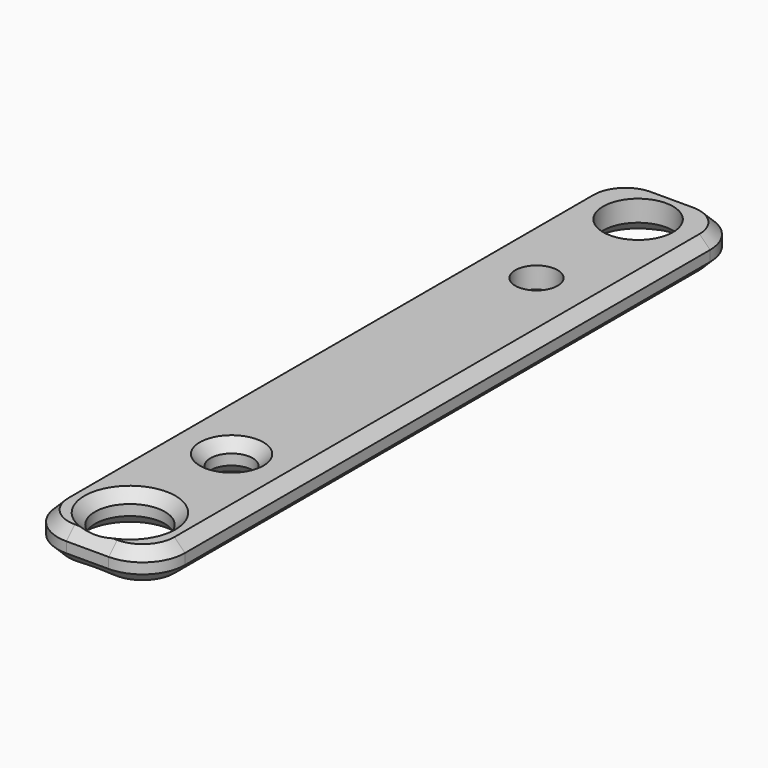
from build123d import *

# Parameters (mm, degrees)
F0_W         = 6
F0_H         = 35
F0_R         = 1.65
F0_R_2       = 1
F1_DEPTH     = 1.5
F2_R         = 2
F3_T1_DEPTH  = 31
F3_T3_DEPTH  = 2
F3_T6_ANGLE  = 90
F3_T8_ANGLE  = 90
F3_T10_ANGLE = 90
F3_T12_ANGLE = 90
F3_T14_ANGLE = 90
F3_T16_ANGLE = 90
F3_T18_ANGLE = 90
F3_T20_ANGLE = 90


# Not quite as in the source:
# - a fillet or chamfer that OpenCascade refuses, or shapes differently, is made with other operations: its cross-section is extruded or revolved along the edge and cut away or added


with BuildPart() as f1:
    # F0 (on Top) → F1 (new body)
    with BuildSketch(Plane.XY):
        Rectangle(F0_W, F0_H)
        with Locations((0.0021975506, -14.9999999195)):
            Circle(F0_R, mode=Mode.SUBTRACT)
        with Locations((0.0021975506, -9)):
            Circle(F0_R_2, mode=Mode.SUBTRACT)
        with Locations((0, 9)):
            Circle(F0_R_2, mode=Mode.SUBTRACT)
        with Locations((0, 15)):
            Circle(F0_R, mode=Mode.SUBTRACT)
    extrude(amount=F1_DEPTH)

    # F2
    f2_edges = [f1.edges().sort_by_distance(p)[0] for p in [
        (-3, 17.5, 0.75),
        (3, 17.5, 0.75),
        (-3, -17.5, 0.75),
        (3, -17.5, 0.75),
    ]]
    fillet(f2_edges, radius=F2_R)

    # F3: chamfer of 0.5 on 22 edges, made by hand

    # F3_s2 → F3_t1 (cut)
    with BuildSketch(Plane.XZ.offset(-15.5)):
        Polygon((-2.5, 1.5), (-3, 1), (-3, 1.5), align=None)
        Polygon((2.5, 1.5), (3, 1), (3, 1.5), align=None)
        Polygon((2.5, 0), (3, 0.5), (3, 0), align=None)
        Polygon((-2.5, 0), (-3, 0.5), (-3, 0), align=None)
    extrude(amount=F3_T1_DEPTH, mode=Mode.SUBTRACT)

    # F3_s4 → F3_t3 (cut)
    with BuildSketch(Plane.YZ.offset(-1)):
        Polygon((17.5, 1), (17, 1.5), (17.5, 1.5), align=None)
        Polygon((-17, 1.5), (-17.5, 1), (-17.5, 1.5), align=None)
        Polygon((17.5, 0.5), (17, 0), (17.5, 0), align=None)
        Polygon((-17, 0), (-17.5, 0.5), (-17.5, 0), align=None)
    extrude(amount=F3_T3_DEPTH, mode=Mode.SUBTRACT)

    # F3_s5 → F3_t6 (revolve, cut)
    with BuildSketch(Plane.YZ.offset(1)):
        Polygon((17.5, 1), (17, 1.5), (17.5, 1.5), align=None)
    revolve(axis=Axis((1, 15.5, 1.5), (0, 0, -1)), revolution_arc=F3_T6_ANGLE, mode=Mode.SUBTRACT)

    # F3_s7 → F3_t8 (revolve, cut)
    with BuildSketch(Plane.YZ.offset(-1)):
        Polygon((17.5, 1), (17, 1.5), (17.5, 1.5), align=None)
    revolve(axis=Axis((-1, 15.5, 1.5), (0, 0, 1)), revolution_arc=F3_T8_ANGLE, mode=Mode.SUBTRACT)

    # F3_s9 → F3_t10 (revolve, cut)
    with BuildSketch(Plane.XZ.offset(15.5)):
        Polygon((-2.5, 1.5), (-3, 1), (-3, 1.5), align=None)
    revolve(axis=Axis((-1, -15.5, 1.5), (0, 0, 1)), revolution_arc=F3_T10_ANGLE, mode=Mode.SUBTRACT)

    # F3_s11 → F3_t12 (revolve, cut)
    with BuildSketch(Plane.YZ.offset(1)):
        Polygon((-17, 1.5), (-17.5, 1), (-17.5, 1.5), align=None)
    revolve(axis=Axis((1, -15.5, 1.5), (0, 0, 1)), revolution_arc=F3_T12_ANGLE, mode=Mode.SUBTRACT)

    # F3_s13 → F3_t14 (revolve, cut)
    with BuildSketch(Plane.YZ.offset(-1)):
        Polygon((17, 0), (17.5, 0.5), (17.5, 0), align=None)
    revolve(axis=Axis((-1, 15.5, 0), (0, 0, 1)), revolution_arc=F3_T14_ANGLE, mode=Mode.SUBTRACT)

    # F3_s15 → F3_t16 (revolve, cut)
    with BuildSketch(Plane.YZ.offset(1)):
        Polygon((17, 0), (17.5, 0.5), (17.5, 0), align=None)
    revolve(axis=Axis((1, 15.5, 0), (0, 0, -1)), revolution_arc=F3_T16_ANGLE, mode=Mode.SUBTRACT)

    # F3_s17 → F3_t18 (revolve, cut)
    with BuildSketch(Plane.XZ.offset(15.5)):
        Polygon((-2.5, 0), (-3, 0.5), (-3, 0), align=None)
    revolve(axis=Axis((-1, -15.5, 0), (0, 0, 1)), revolution_arc=F3_T18_ANGLE, mode=Mode.SUBTRACT)

    # F3_s19 → F3_t20 (revolve, cut)
    with BuildSketch(Plane.YZ.offset(1)):
        Polygon((-17, 0), (-17.5, 0.5), (-17.5, 0), align=None)
    revolve(axis=Axis((1, -15.5, 0), (0, 0, 1)), revolution_arc=F3_T20_ANGLE, mode=Mode.SUBTRACT)

    # F3_s21 → F3_t22 (revolve, cut)
    with BuildSketch(Plane.XZ.offset(9)):
        Polygon((1.5021975506, 0), (1.0021975506, 0.5), (1.0021975506, 0), align=None)
    revolve(axis=Axis((0.0021975506, -9, 0), (0, 0, 1)), mode=Mode.SUBTRACT)

    # F3_s23 → F3_t24 (revolve, cut)
    with BuildSketch(Plane.XZ.offset(-9)):
        Polygon((1.5, 0), (1, 0.5), (1, 0), align=None)
    revolve(axis=Axis((0, 9, 0), (0, 0, 1)), mode=Mode.SUBTRACT)

    # F3_s25 → F3_t26 (revolve, cut)
    with BuildSketch(Plane.XZ.offset(-15)):
        Polygon((2.15, 0), (1.65, 0.5), (1.65, 0), align=None)
    revolve(axis=Axis((0, 15, 0), (0, 0, 1)), mode=Mode.SUBTRACT)

    # F3_s27 → F3_t28 (revolve, cut)
    with BuildSketch(Plane.XZ.offset(9)):
        Polygon((1.5021975506, 1.5), (1.0021975506, 1), (1.0021975506, 1.5), align=None)
    revolve(axis=Axis((0.0021975506, -9, 1.5), (0, 0, 1)), mode=Mode.SUBTRACT)

    # F3_s29 → F3_t30 (revolve, cut)
    with BuildSketch(Plane.XZ.offset(14.9999999195)):
        Polygon((2.1521975506, 1.5), (1.6521975506, 1), (1.6521975506, 1.5), align=None)
    revolve(axis=Axis((0.0021975506, -14.9999999195, 1.5), (0, 0, 1)), mode=Mode.SUBTRACT)

    # F3_s31 → F3_t32 (revolve, cut)
    with BuildSketch(Plane.XZ.offset(14.9999999195)):
        Polygon((2.1521975506, 0), (1.6521975506, 0.5), (1.6521975506, 0), align=None)
    revolve(axis=Axis((0.0021975506, -14.9999999195, 0), (0, 0, 1)), mode=Mode.SUBTRACT)


solid = f1.part
